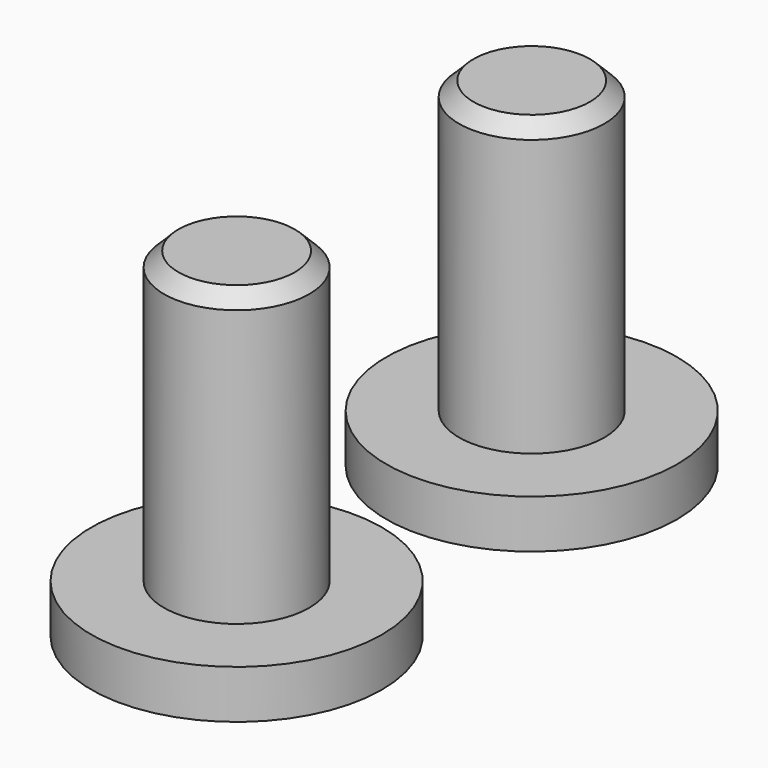
from build123d import *

# Parameters (mm, degrees)
F0_R      = 3
F1_DEPTH  = 1
F2_R      = 1.5
F3_DEPTH  = 6
F4_SIZE   = 0.3
F4_2_SIZE = 0.3


with BuildPart() as f1:
    # F0 (on Top) → F1 (new body)
    with BuildSketch(Plane.XY):
        Circle(F0_R)
    extrude(amount=F1_DEPTH)

    # F2 (on face) → F3 (join)
    with BuildSketch(Plane.XY.offset(1)):
        Circle(F2_R)
    extrude(amount=F3_DEPTH)

    # F4
    f4_edges = [f1.edges().sort_by_distance(p)[0] for p in [
        (-1.5, 0, 7),
    ]]
    chamfer(f4_edges, length=F4_SIZE)


with BuildPart() as f1b:
    # F0 (on Top) → F1, piece 2 (new body)
    with BuildSketch(Plane.XY):
        with Locations((0, 7.61357788)):
            Circle(F0_R)
    extrude(amount=F1_DEPTH)


with BuildPart() as f3:
    # F2 (on face) → F3, piece 2 (new body)
    with BuildSketch(Plane.XY.offset(1)):
        with Locations((0, 7.61357788)):
            Circle(F2_R)
    extrude(amount=F3_DEPTH)

    # F4#2
    f4_2_edges = [f3.edges().sort_by_distance(p)[0] for p in [
        (-1.5, 7.613578, 7),
    ]]
    chamfer(f4_2_edges, length=F4_2_SIZE)


solid = Compound([f1.part, f1b.part, f3.part])
